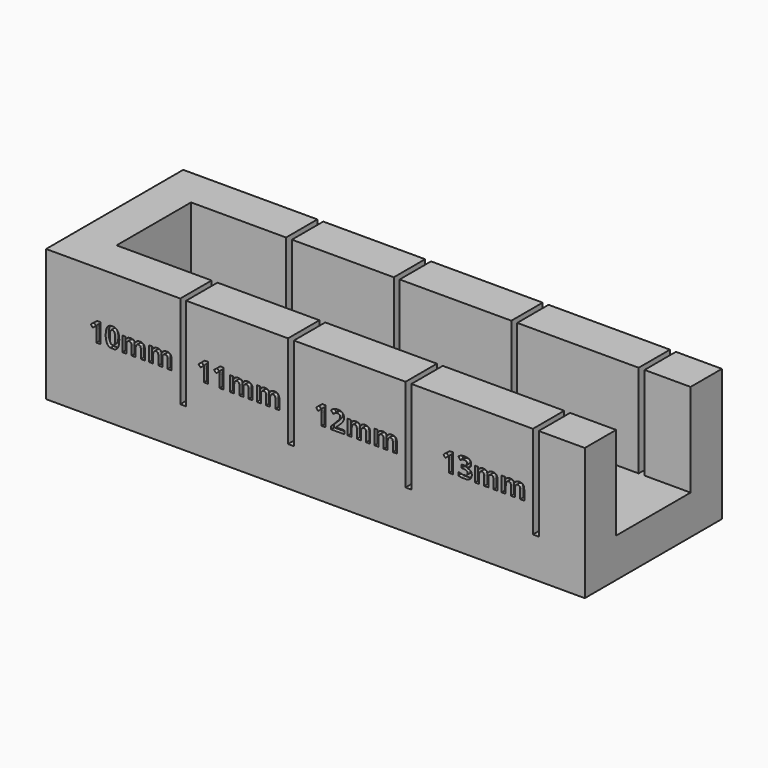
from build123d import *

# Parameters (mm, degrees)
F0_W         = 9.7
F0_H         = 9.5
F0_W_2       = 0.3
F0_W_3       = 10.4
F0_W_4       = 11.4
F0_W_5       = 12.4
F0_W_6       = 4.7
F0_H_2       = 4
F1_DEPTH     = 4
F0_W_7       = 4
F2_DEPTH     = 13.5
F3_TEXT_SIZE = 2.7777777778
F4_DEPTH     = 0.4


# Not quite as in the source:
# - Text() gives the source's letters only with a copy of the font that has no kerning and outlines rounded to 1/6400 em; it was checked with that copy


with BuildPart() as f1:
    # F0 (on Top) → F1 (new body)
    with BuildSketch(Plane.XY):
        with Locations((0.6184425116, -14.4160883874)):
            Rectangle(F0_W, F0_H)
        with Locations((5.6184425116, -14.4160883874)):
            Rectangle(F0_W_2, F0_H)
        with Locations((5.9184425116, -14.4160883874)):
            Rectangle(F0_W_2, F0_H)
        with Locations((11.2684425116, -14.4160883874)):
            Rectangle(F0_W_3, F0_H)
        with Locations((16.6184425116, -14.4160883874)):
            Rectangle(F0_W_2, F0_H)
        with Locations((16.9184425116, -14.4160883874)):
            Rectangle(F0_W_2, F0_H)
        with Locations((22.7684425116, -14.4160883874)):
            Rectangle(F0_W_4, F0_H)
        with Locations((28.6184425116, -14.4160883874)):
            Rectangle(F0_W_2, F0_H)
        with Locations((28.9184425116, -14.4160883874)):
            Rectangle(F0_W_2, F0_H)
        with Locations((35.2684425116, -14.4160883874)):
            Rectangle(F0_W_5, F0_H)
        with Locations((41.6184425116, -14.4160883874)):
            Rectangle(F0_W_2, F0_H)
        with Locations((41.9184425116, -14.4160883874)):
            Rectangle(F0_W_2, F0_H)
        with Locations((44.4184425116, -14.4160883874)):
            Rectangle(F0_W_6, F0_H)
        with Locations((41.9184425116, -7.6660883874)):
            Rectangle(F0_W_2, F0_H_2)
        with Locations((41.6184425116, -7.6660883874)):
            Rectangle(F0_W_2, F0_H_2)
        with Locations((28.9184425116, -7.6660883874)):
            Rectangle(F0_W_2, F0_H_2)
        with Locations((28.6184425116, -7.6660883874)):
            Rectangle(F0_W_2, F0_H_2)
        with Locations((16.9184425116, -7.6660883874)):
            Rectangle(F0_W_2, F0_H_2)
        with Locations((16.6184425116, -7.6660883874)):
            Rectangle(F0_W_2, F0_H_2)
        with Locations((5.9184425116, -7.6660883874)):
            Rectangle(F0_W_2, F0_H_2)
        with Locations((5.6184425116, -7.6660883874)):
            Rectangle(F0_W_2, F0_H_2)
        with Locations((5.6184425116, -21.1660883874)):
            Rectangle(F0_W_2, F0_H_2)
        with Locations((5.9184425116, -21.1660883874)):
            Rectangle(F0_W_2, F0_H_2)
        with Locations((16.6184425116, -21.1660883874)):
            Rectangle(F0_W_2, F0_H_2)
        with Locations((16.9184425116, -21.1660883874)):
            Rectangle(F0_W_2, F0_H_2)
        with Locations((28.6184425116, -21.1660883874)):
            Rectangle(F0_W_2, F0_H_2)
        with Locations((28.9184425116, -21.1660883874)):
            Rectangle(F0_W_2, F0_H_2)
        with Locations((41.6184425116, -21.1660883874)):
            Rectangle(F0_W_2, F0_H_2)
        with Locations((41.9184425116, -21.1660883874)):
            Rectangle(F0_W_2, F0_H_2)
    extrude(amount=F1_DEPTH)

    # F0 (on Top) → F2 (join)
    with BuildSketch(Plane.XY):
        with Locations((-6.2315574884, -7.6660883874)):
            Rectangle(F0_W_7, F0_H_2)
        with Locations((-6.2315574884, -14.4160883874)):
            Rectangle(F0_W_7, F0_H)
        with Locations((-6.2315574884, -21.1660883874)):
            Rectangle(F0_W_7, F0_H_2)
        with Locations((11.2684425116, -21.1660883874)):
            Rectangle(F0_W_3, F0_H_2)
        with Locations((22.7684425116, -21.1660883874)):
            Rectangle(F0_W_4, F0_H_2)
        with Locations((35.2684425116, -21.1660883874)):
            Rectangle(F0_W_5, F0_H_2)
        with Locations((44.4184425116, -21.1660883874)):
            Rectangle(F0_W_6, F0_H_2)
        with Locations((44.4184425116, -7.6660883874)):
            Rectangle(F0_W_6, F0_H_2)
        with Locations((35.2684425116, -7.6660883874)):
            Rectangle(F0_W_5, F0_H_2)
        with Locations((22.7684425116, -7.6660883874)):
            Rectangle(F0_W_4, F0_H_2)
        with Locations((11.2684425116, -7.6660883874)):
            Rectangle(F0_W_3, F0_H_2)
        with Locations((0.6184425116, -7.6660883874)):
            Rectangle(F0_W, F0_H_2)
        with Locations((0.6184425116, -21.1660883874)):
            Rectangle(F0_W, F0_H_2)
    extrude(amount=F2_DEPTH)

    # F3 (on face) → F4 (cut)
    with BuildSketch(Plane.XZ.offset(23.1660883874)):
        with BuildLine():
            Line((-3.1025210301, 7.8975694444), (-3.1025210301, 6.75))
            Line((-3.1025210301, 6.75), (-2.6832501968, 6.75))
            Line((-2.6832501968, 6.75), (-2.6832501968, 8.7330729167))
            Line((-2.6832501968, 8.7330729167), (-3.0278682523, 8.7330729167))
            Line((-3.0278682523, 8.7330729167), (-3.6667571412, 8.2243923611))
            Line((-3.6667571412, 8.2243923611), (-3.4645001968, 7.9722222222))
            Line((-3.4645001968, 7.9722222222), (-3.2366356134, 8.1553819444))
            add(Edge.make_bspline(
                [(-3.0916703357, 8.2921006944), (-3.1958370023, 8.1879340278), (-3.2366356134, 8.1553819444)],
                knots=[0, 0, 0, 1, 1, 1], degree=2))
            Line((-3.0916703357, 8.2921006944), (-3.0981807523, 8.0859375))
            Line((-3.0981807523, 8.0859375), (-3.1025210301, 7.8975694444))
        make_face()
        with BuildLine():
            add(Edge.make_bspline(
                [(-1.6589005879, 6.75), (-1.8532833103, 6.8066179112), (-1.9707935996, 6.98046875)],
                knots=[0.3256694736, 0.3256694736, 0.3256694736, 1, 1, 1], degree=2))
            Line((-1.6589005879, 6.75), (-1.2390000283, 6.75))
            add(Edge.make_bspline(
                [(-0.928909919, 6.9724392361), (-1.0427562215, 6.8053000854), (-1.2390000283, 6.75)],
                knots=[0, 0, 0, 0.6691374514, 0.6691374514, 0.6691374514], degree=2))
            add(Edge.make_bspline(
                [(-0.7587710301, 7.7413194444), (-0.7587710301, 7.2222222222), (-0.928909919, 6.9724392361)],
                knots=[0, 0, 0, 1, 1, 1], degree=2))
            add(Edge.make_bspline(
                [(-0.9343352662, 8.50390625), (-0.7587710301, 8.2434895833), (-0.7587710301, 7.7413194444)],
                knots=[0, 0, 0, 1, 1, 1], degree=2))
            add(Edge.make_bspline(
                [(-1.4532154746, 8.7643229167), (-1.1098995023, 8.7643229167), (-0.9343352662, 8.50390625)],
                knots=[0, 0, 0, 1, 1, 1], degree=2))
            add(Edge.make_bspline(
                [(-1.9753508912, 8.5154079861), (-1.8056460301, 8.7643229167), (-1.4532154746, 8.7643229167)],
                knots=[0, 0, 0, 1, 1, 1], degree=2))
            add(Edge.make_bspline(
                [(-2.1450557523, 7.7413194444), (-2.1450557523, 8.2664930556), (-1.9753508912, 8.5154079861)],
                knots=[0, 0, 0, 1, 1, 1], degree=2))
            add(Edge.make_bspline(
                [(-1.9707935996, 6.98046875), (-2.1450557523, 7.23828125), (-2.1450557523, 7.7413194444)],
                knots=[0, 0, 0, 1, 1, 1], degree=2))
        make_face()
        with BuildLine():
            add(Edge.make_bspline(
                [(-1.7283890857, 7.7413194444), (-1.7283890857, 7.3767361111), (-1.6654550579, 7.21875)],
                knots=[0, 0, 0, 1, 1, 1], degree=2))
            add(Edge.make_bspline(
                [(-1.6648040162, 8.265625), (-1.7283890857, 8.1063368056), (-1.7283890857, 7.7413194444)],
                knots=[0, 0, 0, 1, 1, 1], degree=2))
            add(Edge.make_bspline(
                [(-1.4532154746, 8.4249131944), (-1.6012189468, 8.4249131944), (-1.6648040162, 8.265625)],
                knots=[0, 0, 0, 1, 1, 1], degree=2))
            add(Edge.make_bspline(
                [(-1.2422779746, 8.265625), (-1.3082501968, 8.4249131944), (-1.4532154746, 8.4249131944)],
                knots=[0, 0, 0, 1, 1, 1], degree=2))
            add(Edge.make_bspline(
                [(-1.1763057523, 7.7413194444), (-1.1763057523, 8.1063368056), (-1.2422779746, 8.265625)],
                knots=[0, 0, 0, 1, 1, 1], degree=2))
            add(Edge.make_bspline(
                [(-1.241409919, 7.220703125), (-1.1763057523, 7.3806423611), (-1.1763057523, 7.7413194444)],
                knots=[0, 0, 0, 1, 1, 1], degree=2))
            add(Edge.make_bspline(
                [(-1.4532154746, 7.0607638889), (-1.3065140857, 7.0607638889), (-1.241409919, 7.220703125)],
                knots=[0, 0, 0, 1, 1, 1], degree=2))
            add(Edge.make_bspline(
                [(-1.6654550579, 7.21875), (-1.6025210301, 7.0607638889), (-1.4532154746, 7.0607638889)],
                knots=[0, 0, 0, 1, 1, 1], degree=2))
        make_face(mode=Mode.SUBTRACT)
        with BuildLine():
            Line((-0.4427988079, 8.2664930556), (-0.4427988079, 6.75))
            Line((-0.4427988079, 6.75), (-0.0291703357, 6.75))
            Line((-0.0291703357, 6.75), (-0.0291703357, 7.4635416667))
            add(Edge.make_bspline(
                [(0.0426612616, 7.8472222222), (-0.0291703357, 7.73046875), (-0.0291703357, 7.4635416667)],
                knots=[0, 0, 0, 1, 1, 1], degree=2))
            add(Edge.make_bspline(
                [(0.2733470254, 7.9639756944), (0.1144928588, 7.9639756944), (0.0426612616, 7.8472222222)],
                knots=[0, 0, 0, 1, 1, 1], degree=2))
            add(Edge.make_bspline(
                [(0.4463070949, 7.8819444444), (0.391402581, 7.9639756944), (0.2733470254, 7.9639756944)],
                knots=[0, 0, 0, 1, 1, 1], degree=2))
            add(Edge.make_bspline(
                [(0.5012116088, 7.6358506944), (0.5012116088, 7.7999131944), (0.4463070949, 7.8819444444)],
                knots=[0, 0, 0, 1, 1, 1], degree=2))
            Line((0.5012116088, 7.6358506944), (0.5012116088, 6.75))
            Line((0.5012116088, 6.75), (0.914840081, 6.75))
            Line((0.914840081, 6.75), (0.914840081, 7.5108506944))
            add(Edge.make_bspline(
                [(0.9901439004, 7.85546875), (0.914840081, 7.7469618056), (0.914840081, 7.5108506944)],
                knots=[0, 0, 0, 1, 1, 1], degree=2))
            add(Edge.make_bspline(
                [(1.2173574421, 7.9639756944), (1.0654477199, 7.9639756944), (0.9901439004, 7.85546875)],
                knots=[0, 0, 0, 1, 1, 1], degree=2))
            add(Edge.make_bspline(
                [(1.3903175116, 7.8819444444), (1.3354129977, 7.9639756944), (1.2173574421, 7.9639756944)],
                knots=[0, 0, 0, 1, 1, 1], degree=2))
            add(Edge.make_bspline(
                [(1.4452220254, 7.6358506944), (1.4452220254, 7.7999131944), (1.3903175116, 7.8819444444)],
                knots=[0, 0, 0, 1, 1, 1], degree=2))
            Line((1.4452220254, 7.6358506944), (1.4452220254, 6.75))
            Line((1.4452220254, 6.75), (1.860152581, 6.75))
            Line((1.860152581, 6.75), (1.860152581, 7.7387152778))
            add(Edge.make_bspline(
                [(1.7279911227, 8.1625434028), (1.860152581, 8.0303819444), (1.860152581, 7.7387152778)],
                knots=[0, 0, 0, 1, 1, 1], degree=2))
            add(Edge.make_bspline(
                [(1.3380171643, 8.2947048611), (1.5958296643, 8.2947048611), (1.7279911227, 8.1625434028)],
                knots=[0, 0, 0, 1, 1, 1], degree=2))
            add(Edge.make_bspline(
                [(1.0702220254, 8.2365451389), (1.1887116088, 8.2947048611), (1.3380171643, 8.2947048611)],
                knots=[0, 0, 0, 1, 1, 1], degree=2))
            add(Edge.make_bspline(
                [(0.8905345254, 8.0724826389), (0.9517324421, 8.1783854167), (1.0702220254, 8.2365451389)],
                knots=[0, 0, 0, 1, 1, 1], degree=2))
            Line((0.8905345254, 8.0724826389), (0.8540761921, 8.0724826389))
            add(Edge.make_bspline(
                [(0.3927046643, 8.2947048611), (0.7329824421, 8.2947048611), (0.8540761921, 8.0724826389)],
                knots=[0, 0, 0, 1, 1, 1], degree=2))
            add(Edge.make_bspline(
                [(0.1281647338, 8.2358940972), (0.2433991088, 8.2947048611), (0.3927046643, 8.2947048611)],
                knots=[0, 0, 0, 1, 1, 1], degree=2))
            add(Edge.make_bspline(
                [(-0.0482675579, 8.0724826389), (0.0129303588, 8.1770833333), (0.1281647338, 8.2358940972)],
                knots=[0, 0, 0, 1, 1, 1], degree=2))
            Line((-0.0482675579, 8.0724826389), (-0.0712710301, 8.0724826389))
            Line((-0.0712710301, 8.0724826389), (-0.1268265857, 8.2664930556))
            Line((-0.1268265857, 8.2664930556), (-0.4427988079, 8.2664930556))
        make_face()
        with BuildLine():
            Line((40.172652581, 6.75), (40.5875831366, 6.75))
            Line((40.5875831366, 6.75), (40.5875831366, 7.7387152778))
            add(Edge.make_bspline(
                [(40.4554216782, 8.1625434028), (40.5875831366, 8.0303819444), (40.5875831366, 7.7387152778)],
                knots=[0, 0, 0, 1, 1, 1], degree=2))
            add(Edge.make_bspline(
                [(40.0654477199, 8.2947048611), (40.3232602199, 8.2947048611), (40.4554216782, 8.1625434028)],
                knots=[0, 0, 0, 1, 1, 1], degree=2))
            add(Edge.make_bspline(
                [(39.797652581, 8.2365451389), (39.9161421643, 8.2947048611), (40.0654477199, 8.2947048611)],
                knots=[0, 0, 0, 1, 1, 1], degree=2))
            add(Edge.make_bspline(
                [(39.617965081, 8.0724826389), (39.6791629977, 8.1783854167), (39.797652581, 8.2365451389)],
                knots=[0, 0, 0, 1, 1, 1], degree=2))
            Line((39.617965081, 8.0724826389), (39.5815067477, 8.0724826389))
            add(Edge.make_bspline(
                [(39.1201352199, 8.2947048611), (39.4604129977, 8.2947048611), (39.5815067477, 8.0724826389)],
                knots=[0, 0, 0, 1, 1, 1], degree=2))
            add(Edge.make_bspline(
                [(38.8555952893, 8.2358940972), (38.9708296643, 8.2947048611), (39.1201352199, 8.2947048611)],
                knots=[0, 0, 0, 1, 1, 1], degree=2))
            add(Edge.make_bspline(
                [(38.6791629977, 8.0724826389), (38.7403609143, 8.1770833333), (38.8555952893, 8.2358940972)],
                knots=[0, 0, 0, 1, 1, 1], degree=2))
            Line((38.6791629977, 8.0724826389), (38.6561595254, 8.0724826389))
            Line((38.6561595254, 8.0724826389), (38.6006039699, 8.2664930556))
            Line((38.6006039699, 8.2664930556), (38.2846317477, 8.2664930556))
            Line((38.2846317477, 8.2664930556), (38.2846317477, 6.75))
            Line((38.2846317477, 6.75), (38.6982602199, 6.75))
            Line((38.6982602199, 6.75), (38.6982602199, 7.4635416667))
            add(Edge.make_bspline(
                [(38.7700918171, 7.8472222222), (38.6982602199, 7.73046875), (38.6982602199, 7.4635416667)],
                knots=[0, 0, 0, 1, 1, 1], degree=2))
            add(Edge.make_bspline(
                [(39.000777581, 7.9639756944), (38.8419234143, 7.9639756944), (38.7700918171, 7.8472222222)],
                knots=[0, 0, 0, 1, 1, 1], degree=2))
            add(Edge.make_bspline(
                [(39.1737376504, 7.8819444444), (39.1188331366, 7.9639756944), (39.000777581, 7.9639756944)],
                knots=[0, 0, 0, 1, 1, 1], degree=2))
            add(Edge.make_bspline(
                [(39.2286421643, 7.6358506944), (39.2286421643, 7.7999131944), (39.1737376504, 7.8819444444)],
                knots=[0, 0, 0, 1, 1, 1], degree=2))
            Line((39.2286421643, 7.6358506944), (39.2286421643, 6.75))
            Line((39.2286421643, 6.75), (39.6422706366, 6.75))
            Line((39.6422706366, 6.75), (39.6422706366, 7.5108506944))
            add(Edge.make_bspline(
                [(39.717574456, 7.85546875), (39.6422706366, 7.7469618056), (39.6422706366, 7.5108506944)],
                knots=[0, 0, 0, 1, 1, 1], degree=2))
            add(Edge.make_bspline(
                [(39.9447879977, 7.9639756944), (39.7928782754, 7.9639756944), (39.717574456, 7.85546875)],
                knots=[0, 0, 0, 1, 1, 1], degree=2))
            add(Edge.make_bspline(
                [(40.1177480671, 7.8819444444), (40.0628435532, 7.9639756944), (39.9447879977, 7.9639756944)],
                knots=[0, 0, 0, 1, 1, 1], degree=2))
            add(Edge.make_bspline(
                [(40.172652581, 7.6358506944), (40.172652581, 7.7999131944), (40.1177480671, 7.8819444444)],
                knots=[0, 0, 0, 1, 1, 1], degree=2))
            Line((40.172652581, 7.6358506944), (40.172652581, 6.75))
        make_face()
        with BuildLine():
            Line((37.4452220254, 6.75), (37.860152581, 6.75))
            Line((37.860152581, 6.75), (37.860152581, 7.7387152778))
            add(Edge.make_bspline(
                [(37.7279911227, 8.1625434028), (37.860152581, 8.0303819444), (37.860152581, 7.7387152778)],
                knots=[0, 0, 0, 1, 1, 1], degree=2))
            add(Edge.make_bspline(
                [(37.3380171643, 8.2947048611), (37.5958296643, 8.2947048611), (37.7279911227, 8.1625434028)],
                knots=[0, 0, 0, 1, 1, 1], degree=2))
            add(Edge.make_bspline(
                [(37.0702220254, 8.2365451389), (37.1887116088, 8.2947048611), (37.3380171643, 8.2947048611)],
                knots=[0, 0, 0, 1, 1, 1], degree=2))
            add(Edge.make_bspline(
                [(36.8905345254, 8.0724826389), (36.9517324421, 8.1783854167), (37.0702220254, 8.2365451389)],
                knots=[0, 0, 0, 1, 1, 1], degree=2))
            Line((36.8905345254, 8.0724826389), (36.8540761921, 8.0724826389))
            add(Edge.make_bspline(
                [(36.3927046643, 8.2947048611), (36.7329824421, 8.2947048611), (36.8540761921, 8.0724826389)],
                knots=[0, 0, 0, 1, 1, 1], degree=2))
            add(Edge.make_bspline(
                [(36.1281647338, 8.2358940972), (36.2433991088, 8.2947048611), (36.3927046643, 8.2947048611)],
                knots=[0, 0, 0, 1, 1, 1], degree=2))
            add(Edge.make_bspline(
                [(35.9517324421, 8.0724826389), (36.0129303588, 8.1770833333), (36.1281647338, 8.2358940972)],
                knots=[0, 0, 0, 1, 1, 1], degree=2))
            Line((35.9517324421, 8.0724826389), (35.9287289699, 8.0724826389))
            Line((35.9287289699, 8.0724826389), (35.8731734143, 8.2664930556))
            Line((35.8731734143, 8.2664930556), (35.5572011921, 8.2664930556))
            Line((35.5572011921, 8.2664930556), (35.5572011921, 6.75))
            Line((35.5572011921, 6.75), (35.9708296643, 6.75))
            Line((35.9708296643, 6.75), (35.9708296643, 7.4635416667))
            add(Edge.make_bspline(
                [(36.0426612616, 7.8472222222), (35.9708296643, 7.73046875), (35.9708296643, 7.4635416667)],
                knots=[0, 0, 0, 1, 1, 1], degree=2))
            add(Edge.make_bspline(
                [(36.2733470254, 7.9639756944), (36.1144928588, 7.9639756944), (36.0426612616, 7.8472222222)],
                knots=[0, 0, 0, 1, 1, 1], degree=2))
            add(Edge.make_bspline(
                [(36.4463070949, 7.8819444444), (36.391402581, 7.9639756944), (36.2733470254, 7.9639756944)],
                knots=[0, 0, 0, 1, 1, 1], degree=2))
            add(Edge.make_bspline(
                [(36.5012116088, 7.6358506944), (36.5012116088, 7.7999131944), (36.4463070949, 7.8819444444)],
                knots=[0, 0, 0, 1, 1, 1], degree=2))
            Line((36.5012116088, 7.6358506944), (36.5012116088, 6.75))
            Line((36.5012116088, 6.75), (36.914840081, 6.75))
            Line((36.914840081, 6.75), (36.914840081, 7.5108506944))
            add(Edge.make_bspline(
                [(36.9901439004, 7.85546875), (36.914840081, 7.7469618056), (36.914840081, 7.5108506944)],
                knots=[0, 0, 0, 1, 1, 1], degree=2))
            add(Edge.make_bspline(
                [(37.2173574421, 7.9639756944), (37.0654477199, 7.9639756944), (36.9901439004, 7.85546875)],
                knots=[0, 0, 0, 1, 1, 1], degree=2))
            add(Edge.make_bspline(
                [(37.3903175116, 7.8819444444), (37.3354129977, 7.9639756944), (37.2173574421, 7.9639756944)],
                knots=[0, 0, 0, 1, 1, 1], degree=2))
            add(Edge.make_bspline(
                [(37.4452220254, 7.6358506944), (37.4452220254, 7.7999131944), (37.3903175116, 7.8819444444)],
                knots=[0, 0, 0, 1, 1, 1], degree=2))
            Line((37.4452220254, 7.6358506944), (37.4452220254, 6.75))
        make_face()
        with BuildLine():
            Line((32.8974789699, 7.8975694444), (32.8974789699, 6.75))
            Line((32.8974789699, 6.75), (33.3167498032, 6.75))
            Line((33.3167498032, 6.75), (33.3167498032, 8.7330729167))
            Line((33.3167498032, 8.7330729167), (32.9721317477, 8.7330729167))
            Line((32.9721317477, 8.7330729167), (32.3332428588, 8.2243923611))
            Line((32.3332428588, 8.2243923611), (32.5354998032, 7.9722222222))
            Line((32.5354998032, 7.9722222222), (32.7633643866, 8.1553819444))
            add(Edge.make_bspline(
                [(32.9083296643, 8.2921006944), (32.8041629977, 8.1879340278), (32.7633643866, 8.1553819444)],
                knots=[0, 0, 0, 1, 1, 1], degree=2))
            Line((32.9083296643, 8.2921006944), (32.9018192477, 8.0859375))
            Line((32.9018192477, 8.0859375), (32.8974789699, 7.8975694444))
        make_face()
        with BuildLine():
            Line((4.172652581, 6.75), (4.5875831366, 6.75))
            Line((4.5875831366, 6.75), (4.5875831366, 7.7387152778))
            add(Edge.make_bspline(
                [(4.4554216782, 8.1625434028), (4.5875831366, 8.0303819444), (4.5875831366, 7.7387152778)],
                knots=[0, 0, 0, 1, 1, 1], degree=2))
            add(Edge.make_bspline(
                [(4.0654477199, 8.2947048611), (4.3232602199, 8.2947048611), (4.4554216782, 8.1625434028)],
                knots=[0, 0, 0, 1, 1, 1], degree=2))
            add(Edge.make_bspline(
                [(3.797652581, 8.2365451389), (3.9161421643, 8.2947048611), (4.0654477199, 8.2947048611)],
                knots=[0, 0, 0, 1, 1, 1], degree=2))
            add(Edge.make_bspline(
                [(3.617965081, 8.0724826389), (3.6791629977, 8.1783854167), (3.797652581, 8.2365451389)],
                knots=[0, 0, 0, 1, 1, 1], degree=2))
            Line((3.617965081, 8.0724826389), (3.5815067477, 8.0724826389))
            add(Edge.make_bspline(
                [(3.1201352199, 8.2947048611), (3.4604129977, 8.2947048611), (3.5815067477, 8.0724826389)],
                knots=[0, 0, 0, 1, 1, 1], degree=2))
            add(Edge.make_bspline(
                [(2.8555952893, 8.2358940972), (2.9708296643, 8.2947048611), (3.1201352199, 8.2947048611)],
                knots=[0, 0, 0, 1, 1, 1], degree=2))
            add(Edge.make_bspline(
                [(2.6791629977, 8.0724826389), (2.7403609143, 8.1770833333), (2.8555952893, 8.2358940972)],
                knots=[0, 0, 0, 1, 1, 1], degree=2))
            Line((2.6791629977, 8.0724826389), (2.6561595254, 8.0724826389))
            Line((2.6561595254, 8.0724826389), (2.6006039699, 8.2664930556))
            Line((2.6006039699, 8.2664930556), (2.2846317477, 8.2664930556))
            Line((2.2846317477, 8.2664930556), (2.2846317477, 6.75))
            Line((2.2846317477, 6.75), (2.6982602199, 6.75))
            Line((2.6982602199, 6.75), (2.6982602199, 7.4635416667))
            add(Edge.make_bspline(
                [(2.7700918171, 7.8472222222), (2.6982602199, 7.73046875), (2.6982602199, 7.4635416667)],
                knots=[0, 0, 0, 1, 1, 1], degree=2))
            add(Edge.make_bspline(
                [(3.000777581, 7.9639756944), (2.8419234143, 7.9639756944), (2.7700918171, 7.8472222222)],
                knots=[0, 0, 0, 1, 1, 1], degree=2))
            add(Edge.make_bspline(
                [(3.1737376504, 7.8819444444), (3.1188331366, 7.9639756944), (3.000777581, 7.9639756944)],
                knots=[0, 0, 0, 1, 1, 1], degree=2))
            add(Edge.make_bspline(
                [(3.2286421643, 7.6358506944), (3.2286421643, 7.7999131944), (3.1737376504, 7.8819444444)],
                knots=[0, 0, 0, 1, 1, 1], degree=2))
            Line((3.2286421643, 7.6358506944), (3.2286421643, 6.75))
            Line((3.2286421643, 6.75), (3.6422706366, 6.75))
            Line((3.6422706366, 6.75), (3.6422706366, 7.5108506944))
            add(Edge.make_bspline(
                [(3.717574456, 7.85546875), (3.6422706366, 7.7469618056), (3.6422706366, 7.5108506944)],
                knots=[0, 0, 0, 1, 1, 1], degree=2))
            add(Edge.make_bspline(
                [(3.9447879977, 7.9639756944), (3.7928782754, 7.9639756944), (3.717574456, 7.85546875)],
                knots=[0, 0, 0, 1, 1, 1], degree=2))
            add(Edge.make_bspline(
                [(4.1177480671, 7.8819444444), (4.0628435532, 7.9639756944), (3.9447879977, 7.9639756944)],
                knots=[0, 0, 0, 1, 1, 1], degree=2))
            add(Edge.make_bspline(
                [(4.172652581, 7.6358506944), (4.172652581, 7.7999131944), (4.1177480671, 7.8819444444)],
                knots=[0, 0, 0, 1, 1, 1], degree=2))
            Line((4.172652581, 7.6358506944), (4.172652581, 6.75))
        make_face()
        with Locations((7.1691803588, 6.75)):
            Text('11mm', F3_TEXT_SIZE, font='Open Sans', font_style=FontStyle.BOLD, text_align=(TextAlign.LEFT, TextAlign.BOTTOM))
        with Locations((19.1691803588, 6.75)):
            Text('12mm', F3_TEXT_SIZE, font='Open Sans', font_style=FontStyle.BOLD, text_align=(TextAlign.LEFT, TextAlign.BOTTOM))
        with BuildLine():
            add(Edge.make_bspline(
                [(34.1256094504, 6.75), (33.9841129369, 6.7767984971), (33.8605866088, 6.8298611111)],
                knots=[0.5050353738, 0.5050353738, 0.5050353738, 1, 1, 1], degree=2))
            Line((34.1256094504, 6.75), (34.7214336121, 6.75))
            add(Edge.make_bspline(
                [(35.0255171643, 6.8821614583), (34.9039506723, 6.7886976805), (34.7214336121, 6.75)],
                knots=[0, 0, 0, 0.5859606644, 0.5859606644, 0.5859606644], degree=2))
            add(Edge.make_bspline(
                [(35.2329824421, 7.3276909722), (35.2329824421, 7.0416666667), (35.0255171643, 6.8821614583)],
                knots=[0, 0, 0, 1, 1, 1], degree=2))
            add(Edge.make_bspline(
                [(35.1097185532, 7.6404079861), (35.2329824421, 7.5243055556), (35.2329824421, 7.3276909722)],
                knots=[0, 0, 0, 1, 1, 1], degree=2))
            add(Edge.make_bspline(
                [(34.7460032754, 7.7864583333), (34.9864546643, 7.7565104167), (35.1097185532, 7.6404079861)],
                knots=[0, 0, 0, 1, 1, 1], degree=2))
            Line((34.7460032754, 7.7864583333), (34.7460032754, 7.7942708333))
            add(Edge.make_bspline(
                [(35.0621925116, 7.9735243056), (34.9495623032, 7.8433159722), (34.7460032754, 7.7942708333)],
                knots=[0, 0, 0, 1, 1, 1], degree=2))
            add(Edge.make_bspline(
                [(35.1748227199, 8.2894965278), (35.1748227199, 8.1037326389), (35.0621925116, 7.9735243056)],
                knots=[0, 0, 0, 1, 1, 1], degree=2))
            add(Edge.make_bspline(
                [(34.9964373032, 8.6365017361), (35.1748227199, 8.51171875), (35.1748227199, 8.2894965278)],
                knots=[0, 0, 0, 1, 1, 1], degree=2))
            add(Edge.make_bspline(
                [(34.5103261921, 8.7612847222), (34.8180518866, 8.7612847222), (34.9964373032, 8.6365017361)],
                knots=[0, 0, 0, 1, 1, 1], degree=2))
            add(Edge.make_bspline(
                [(33.8631907754, 8.5659722222), (34.1344581366, 8.7612847222), (34.5103261921, 8.7612847222)],
                knots=[0, 0, 0, 1, 1, 1], degree=2))
            Line((33.8631907754, 8.5659722222), (34.0572011921, 8.27734375))
            add(Edge.make_bspline(
                [(34.2815935532, 8.3897569444), (34.180465081, 8.3572048611), (34.0572011921, 8.27734375)],
                knots=[0, 0, 0, 1, 1, 1], degree=2))
            add(Edge.make_bspline(
                [(34.4803782754, 8.4223090278), (34.3827220254, 8.4223090278), (34.2815935532, 8.3897569444)],
                knots=[0, 0, 0, 1, 1, 1], degree=2))
            add(Edge.make_bspline(
                [(34.762496331, 8.1970486111), (34.762496331, 8.4223090278), (34.4803782754, 8.4223090278)],
                knots=[0, 0, 0, 1, 1, 1], degree=2))
            add(Edge.make_bspline(
                [(34.6559425116, 7.9904513889), (34.762496331, 8.05078125), (34.762496331, 8.1970486111)],
                knots=[0, 0, 0, 1, 1, 1], degree=2))
            add(Edge.make_bspline(
                [(34.3189199421, 7.9301215278), (34.5493886921, 7.9301215278), (34.6559425116, 7.9904513889)],
                knots=[0, 0, 0, 1, 1, 1], degree=2))
            Line((34.3189199421, 7.9301215278), (34.1657081366, 7.9301215278))
            Line((34.1657081366, 7.9301215278), (34.1657081366, 7.6085069444))
            Line((34.1657081366, 7.6085069444), (34.3163157754, 7.6085069444))
            add(Edge.make_bspline(
                [(34.6798140393, 7.5501302083), (34.5658817477, 7.6085069444), (34.3163157754, 7.6085069444)],
                knots=[0, 0, 0, 1, 1, 1], degree=2))
            add(Edge.make_bspline(
                [(34.793746331, 7.3524305556), (34.793746331, 7.4917534722), (34.6798140393, 7.5501302083)],
                knots=[0, 0, 0, 1, 1, 1], degree=2))
            add(Edge.make_bspline(
                [(34.6947879977, 7.1256510417), (34.793746331, 7.1961805556), (34.793746331, 7.3524305556)],
                knots=[0, 0, 0, 1, 1, 1], degree=2))
            add(Edge.make_bspline(
                [(34.3879303588, 7.0551215278), (34.5958296643, 7.0551215278), (34.6947879977, 7.1256510417)],
                knots=[0, 0, 0, 1, 1, 1], degree=2))
            add(Edge.make_bspline(
                [(34.114058831, 7.091796875), (34.2525136921, 7.0551215278), (34.3879303588, 7.0551215278)],
                knots=[0, 0, 0, 1, 1, 1], degree=2))
            add(Edge.make_bspline(
                [(33.8605866088, 7.1866319444), (33.9756039699, 7.1284722222), (34.114058831, 7.091796875)],
                knots=[0, 0, 0, 1, 1, 1], degree=2))
            Line((33.8605866088, 7.1866319444), (33.8605866088, 6.8298611111))
        make_face()
    extrude(amount=-F4_DEPTH, mode=Mode.SUBTRACT)


solid = f1.part
